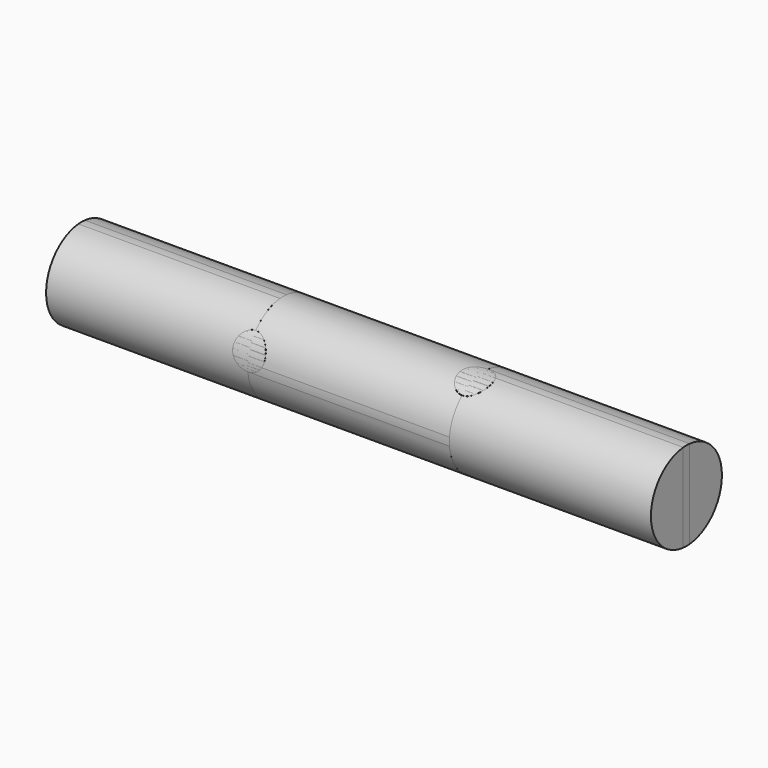
from build123d import *

# Parameters (mm, degrees)
F0_W     = 25
F0_H     = 9.5
F1_DEPTH = 10
F2_DEPTH = 10
F5_ANGLE = 90
F6_R     = 2
F7_DEPTH = 20
F9_ANGLE = 90
F10_W    = 77
F10_H    = 5.5


with BuildPart() as f1:
    # F0 (on Top) → F1 (new body, symmetric)
    with BuildSketch(Plane.XY):
        with Locations((12.5, -5.25)):
            Rectangle(F0_W, F0_H)
    extrude(amount=F1_DEPTH, both=True)


with BuildPart() as f1b:
    # F0 (on Top) → F1, piece 2 (new body, symmetric)
    with BuildSketch(Plane.XY):
        with Locations((12.5, 5.25)):
            Rectangle(F0_W, F0_H)
    extrude(amount=F1_DEPTH, both=True)


with BuildPart() as f2:
    # F0 (on Top) → F2 (new body, symmetric)
    with BuildSketch(Plane.XY):
        Polygon((0, 0.5), (0, 0), (0, -0.5), (25, -0.5), (25, 0.5), align=None)
    extrude(amount=F2_DEPTH, both=True)


with BuildPart() as f3_1:
    # F3: copy of F1
    add(f1.part.moved(Location((25, 0, 0))))


with BuildPart() as f3_2:
    # F3: copy of F1b
    add(f1b.part.moved(Location((25, 0, 0))))


with BuildPart() as f3_3:
    # F3: copy of F2
    add(f2.part.moved(Location((25, 0, 0))))


with BuildPart() as f3_2_1:
    # F5: moved
    add(f3_2.part.rotate(Axis((36.7808852345, 0, 0), (1, 0, 0)), F5_ANGLE))


with BuildPart() as f3_3_1:
    # F5: moved
    add(f3_3.part.rotate(Axis((36.7808852345, 0, 0), (1, 0, 0)), F5_ANGLE))


with BuildPart() as f3_1_1:
    # F5: moved
    add(f3_1.part.rotate(Axis((36.7808852345, 0, 0), (1, 0, 0)), F5_ANGLE))


with BuildPart() as f7:
    # F6 (on face) → F7 (new body)
    with BuildSketch(Plane.XZ.offset(10)):
        with Locations((25, 1.5)):
            Circle(F6_R)
    extrude(amount=-F7_DEPTH)


with BuildPart() as f8_1:
    # F8: copy of F3_2
    add(f3_2_1.part.moved(Location((25, 0, 0))))


with BuildPart() as f8_2:
    # F8: copy of F3_3
    add(f3_3_1.part.moved(Location((25, 0, 0))))


with BuildPart() as f8_3:
    # F8: copy of F3_1
    add(f3_1_1.part.moved(Location((25, 0, 0))))


with BuildPart() as f8_4:
    # F8: copy of F7
    add(f7.part.moved(Location((25, 0, 0))))


with BuildPart() as f8_4_1:
    # F9: moved
    add(f8_4.part.rotate(Axis((36.7808852345, 0, 0), (1, 0, 0)), F9_ANGLE))


with BuildPart() as f8_1_1:
    # F9: moved
    add(f8_1.part.rotate(Axis((36.7808852345, 0, 0), (1, 0, 0)), F9_ANGLE))


with BuildPart() as f8_2_1:
    # F9: moved
    add(f8_2.part.rotate(Axis((36.7808852345, 0, 0), (1, 0, 0)), F9_ANGLE))


with BuildPart() as f8_3_1:
    # F9: moved
    add(f8_3.part.rotate(Axis((36.7808852345, 0, 0), (1, 0, 0)), F9_ANGLE))


with BuildPart() as f11_tool:
    # F10 (on Front) → F11 (revolve)
    with BuildSketch(Plane.XZ):
        with Locations((38.5, 2.75)):
            Rectangle(F10_W, F10_H)
    revolve(axis=Axis((36.7808852345, 0, 0), (1, 0, 0)))


with BuildPart() as f1_1:
    add(f1.part)

    # F11: intersect by f11_tool
    add(f11_tool.part, mode=Mode.INTERSECT)


with BuildPart() as f1b_1:
    add(f1b.part)

    # F11: intersect by f11_tool
    add(f11_tool.part, mode=Mode.INTERSECT)


with BuildPart() as f2_1:
    add(f2.part)

    # F11: intersect by f11_tool
    add(f11_tool.part, mode=Mode.INTERSECT)


with BuildPart() as f3_1_2:
    add(f3_1_1.part)

    # F11: intersect by f11_tool
    add(f11_tool.part, mode=Mode.INTERSECT)


with BuildPart() as f3_2_2:
    add(f3_2_1.part)

    # F11: intersect by f11_tool
    add(f11_tool.part, mode=Mode.INTERSECT)


with BuildPart() as f3_3_2:
    add(f3_3_1.part)

    # F11: intersect by f11_tool
    add(f11_tool.part, mode=Mode.INTERSECT)


with BuildPart() as f7_1:
    add(f7.part)

    # F11: intersect by f11_tool
    add(f11_tool.part, mode=Mode.INTERSECT)


with BuildPart() as f8_1_2:
    add(f8_1_1.part)

    # F11: intersect by f11_tool
    add(f11_tool.part, mode=Mode.INTERSECT)


with BuildPart() as f8_2_2:
    add(f8_2_1.part)

    # F11: intersect by f11_tool
    add(f11_tool.part, mode=Mode.INTERSECT)


with BuildPart() as f8_3_2:
    add(f8_3_1.part)

    # F11: intersect by f11_tool
    add(f11_tool.part, mode=Mode.INTERSECT)


with BuildPart() as f8_4_2:
    add(f8_4_1.part)

    # F11: intersect by f11_tool
    add(f11_tool.part, mode=Mode.INTERSECT)


solid = Compound([f1_1.part, f1b_1.part, f2_1.part, f3_1_2.part, f3_2_2.part, f3_3_2.part, f7_1.part, f8_1_2.part, f8_2_2.part, f8_3_2.part, f8_4_2.part])
